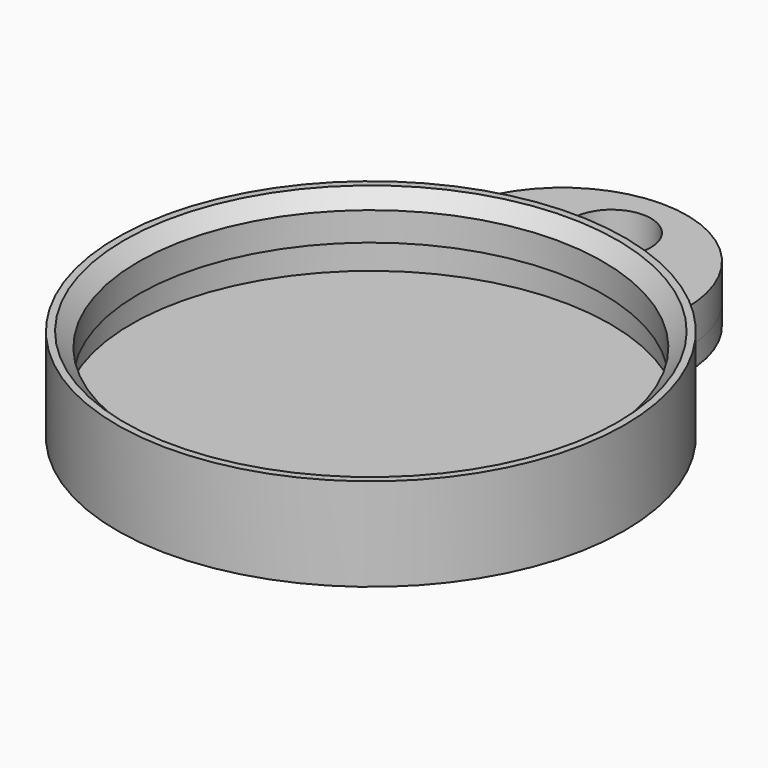
from build123d import *

# Parameters (mm, degrees)
F0_R     = 2.75
F1_DEPTH = 1.5
F2_R     = 16.75
F3_DEPTH = 2
F2_R_2   = 2.75
F5_DEPTH = 2.5
F6_R     = 16.75
F6_R_2   = 16.25
F7_DEPTH = 3
F8_SIZE  = 1
F9_R     = 0.5


# Not quite as in the source:
# - a feature names something its author has since deleted; it is built from what else it names


with BuildPart() as f1:
    # F0 (on Top) → F1 (new body)
    with BuildSketch(Plane.XY):
        with BuildLine():
            ThreePointArc((-8.6418314576, 15.5042332625), (-8.9908284276, -15.3044929412), (17.75, 0))
            ThreePointArc((17.75, 0), (15.3044929412, 8.9908284276), (8.6418314576, 15.5042332625))
            ThreePointArc((8.6418314576, 15.5042332625), (0, 17.75), (-8.6418314576, 15.5042332625))
        make_face()
        with BuildLine():
            ThreePointArc((-8.6418314576, 15.5042332625), (0, 17.75), (8.6418314576, 15.5042332625))
            ThreePointArc((8.6418314576, 15.5042332625), (6.5916833801, 22.4532341762), (0, 25.4601314234))
            ThreePointArc((0, 25.4601314234), (-6.5916833801, 22.4532341762), (-8.6418314576, 15.5042332625))
        make_face()
        with Locations((0, 21.05)):
            Circle(F0_R, mode=Mode.SUBTRACT)
    extrude(amount=F1_DEPTH)

    # F2 (on face) → F3 (join)
    with BuildSketch(Plane.XY.offset(1.5)):
        with BuildLine():
            ThreePointArc((-8.6418314576, 15.5042332625), (-8.9908284276, -15.3044929412), (17.75, 0))
            ThreePointArc((17.75, 0), (15.3044929412, 8.9908284276), (8.6418314576, 15.5042332625))
            ThreePointArc((8.6418314576, 15.5042332625), (0, 17.75), (-8.6418314576, 15.5042332625))
        make_face()
        Circle(F2_R, mode=Mode.SUBTRACT)
    extrude(amount=F3_DEPTH)

    # F2 (on face) → F5 (join)
    with BuildSketch(Plane.XY.offset(1.5)):
        with BuildLine():
            ThreePointArc((-8.6418314576, 15.5042332625), (0, 17.75), (8.6418314576, 15.5042332625))
            ThreePointArc((8.6418314576, 15.5042332625), (0, 25.4601314234), (-8.6418314576, 15.5042332625))
        make_face()
        with Locations((0, 21.05)):
            Circle(F2_R_2, mode=Mode.SUBTRACT)
    extrude(amount=F5_DEPTH)

    # F6 (on face) → F7 (join)
    with BuildSketch(Plane.XY.offset(3.5)):
        with BuildLine():
            ThreePointArc((-8.6418314576, 15.5042332625), (-8.9908284276, -15.3044929412), (17.75, 0))
            ThreePointArc((17.75, 0), (15.3044929412, 8.9908284276), (8.6418314576, 15.5042332625))
            ThreePointArc((8.6418314576, 15.5042332625), (0, 17.75), (-8.6418314576, 15.5042332625))
        make_face()
        Circle(F6_R, mode=Mode.SUBTRACT)
        Circle(F6_R)
        Circle(F6_R_2, mode=Mode.SUBTRACT)
    extrude(amount=F7_DEPTH)

    # F8
    f8_edges = [f1.edges().sort_by_distance(p)[0] for p in [
        (-16.25, 0, 6.5),
    ]]
    chamfer(f8_edges, length=F8_SIZE)

    # F9
    f9_edges = [f1.edges().sort_by_distance(p)[0] for p in [
        (-2.75, 21.05, 0),
    ]]
    fillet(f9_edges, radius=F9_R)


solid = f1.part
